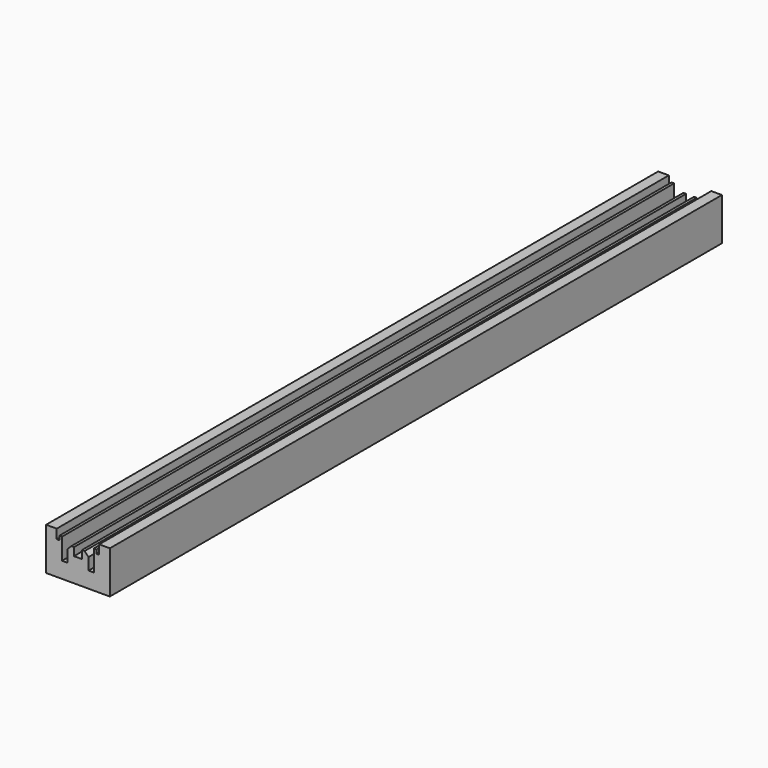
from build123d import *

# Parameters (mm, degrees)
F0_W         = 76.2
F0_H         = 50.8
F1_DEPTH     = 914.4
F2_W         = 50.8
F2_H         = 6.35
F3_DEPTH     = 914.401
F5_DEPTH     = 914.401
F6_W         = 3.175
F6_H         = 4.7625
F7_DEPTH     = 914.401
F9_D         = 6.35
F10_D        = 6.35
F11_T1_DEPTH = 916.7694673581
F11_T3_DEPTH = 40.4694673581


# Not quite as in the source:
# - a fillet or chamfer that OpenCascade refuses, or shapes differently, is made with other operations: its cross-section is extruded or revolved along the edge and cut away or added


with BuildPart() as f1:
    # F0 (on Front) → F1 (new body)
    with BuildSketch(Plane.XZ):
        with Locations((0, -25.4)):
            Rectangle(F0_W, F0_H)
    extrude(amount=F1_DEPTH)

    # F2 (on Front) → F3 (cut, through all)
    with BuildSketch(Plane.XZ):
        with Locations((0, -3.175)):
            Rectangle(F2_W, F2_H)
    extrude(amount=F3_DEPTH, mode=Mode.SUBTRACT)

    # F4 (on Front) → F5 (cut, through all)
    with BuildSketch(Plane.XZ):
        Polygon((0, -6.35), (-19.05, -6.35), (-19.05, -31.75), (-12.7, -31.75), (-12.7, -12.7), (-4.7625, -12.7), (-4.7625, -22.225), (0, -22.225), (4.7625, -22.225), (4.7625, -12.7), (12.7, -12.7), (12.7, -31.75), (19.05, -31.75), (19.05, -6.35), align=None)
    extrude(amount=F5_DEPTH, mode=Mode.SUBTRACT)

    # F6 (on Front) → F7 (cut, through all)
    with BuildSketch(Plane.XZ):
        with Locations((-23.8125, -8.73125)):
            Rectangle(F6_W, F6_H)
        with Locations((23.8125, -8.73125)):
            Rectangle(F6_W, F6_H)
    extrude(amount=F7_DEPTH, mode=Mode.SUBTRACT)

    # F9 (through all)
    with Locations(Plane(origin=(0, 0, -50.8), x_dir=(1, 0, 0), z_dir=(0, 0, -1))):
        with Locations((0, 38.1)):
            Hole(F9_D / 2)

    # F10 (through all)
    with Locations(Plane(origin=(0, 0, -50.8), x_dir=(1, 0, 0), z_dir=(0, 0, -1))):
        with Locations((-13.4874, 19.05), (13.4874, 19.05)):
            Hole(F10_D / 2)

    # F11: chamfer of 4.7625 on 4 edges, made by hand

    # F11_s2 → F11_t1 (cut)
    with BuildSketch(Plane.XZ.offset(9.8781728721)):
        Polygon((-7.9375, -12.7), (-12.7, -17.4625), (-12.7, -12.7), align=None)
        Polygon((7.9375, -12.7), (12.7, -17.4625), (12.7, -12.7), align=None)
    extrude(amount=F11_T1_DEPTH, mode=Mode.SUBTRACT)

    # F11_s4 → F11_t3 (cut)
    with BuildSketch(Plane.XZ.offset(-12.2476402302)):
        Polygon((12.7, -17.4625), (7.9375, -12.7), (12.7, -12.7), align=None)
        Polygon((-7.9375, -12.7), (-12.7, -17.4625), (-12.7, -12.7), align=None)
    extrude(amount=F11_T3_DEPTH, mode=Mode.SUBTRACT)


solid = f1.part
